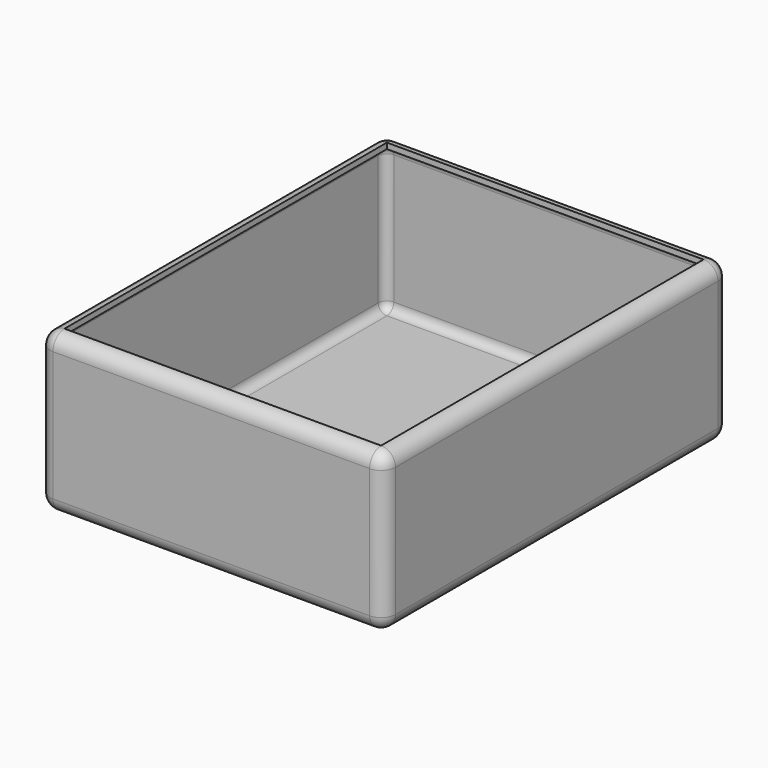
from build123d import *

# Parameters (mm, degrees)
F1_DEPTH = 55
F2_R     = 5
F3_T     = -2


# Not quite as in the source:
# - a shell that OpenCascade refuses in one call is made with other operations: the cavity is built on its own and cut out


with BuildPart() as f1:
    # F0 (on Top) → F1 (new body)
    with BuildSketch(Plane.XY):
        with BuildLine():
            Line((-55, -75), (55, -75))
            ThreePointArc((55, -75), (58.5355339059, -73.5355339059), (60, -70))
            Line((60, -70), (60, 70))
            ThreePointArc((60, 70), (58.5355339059, 73.5355339059), (55, 75))
            Line((55, 75), (-55, 75))
            ThreePointArc((-55, 75), (-58.5355339059, 73.5355339059), (-60, 70))
            Line((-60, 70), (-60, -70))
            ThreePointArc((-60, -70), (-58.5355339059, -73.5355339059), (-55, -75))
        make_face()
    extrude(amount=F1_DEPTH)

    # F2
    f2_edges = [f1.edges().sort_by_distance(p)[0] for p in [
        (-60, 0, 55),
        (-60, 0, 0),
    ]]
    fillet(f2_edges, radius=F2_R)

    # F3: a shell. OpenCascade refuses it in one call, so the cavity is built on its own and cut out:
    # the body offset inwards by the wall thickness, plus a prism from it out through each open face.
    f3_core = offset(f1.part, amount=F3_T, mode=Mode.PRIVATE)
    f3_exits = [f3_core.faces().sort_by_distance(p)[0] for p in [
        (0, 0, 53),
    ]]
    add(f3_core, mode=Mode.SUBTRACT)
    extrude(f3_exits, amount=-F3_T, mode=Mode.SUBTRACT)


solid = f1.part
